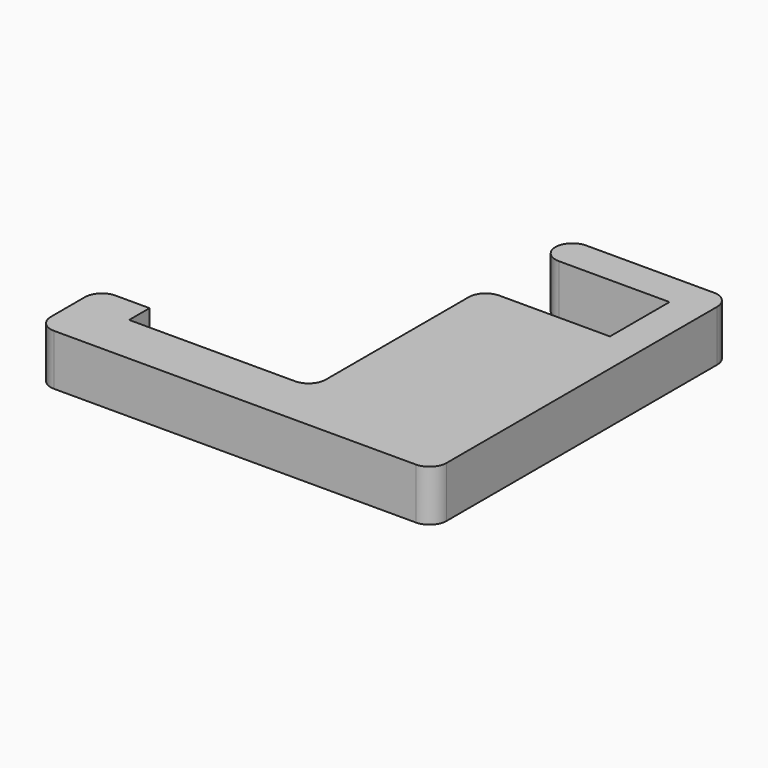
from build123d import *

# Parameters (mm, degrees)
F1_DEPTH = 12
F2_R     = 3.99999


# Not quite as in the source:
# - a fillet or chamfer is up to 0.001 mm smaller than in the source, because OpenCascade refuses the exact size
# - a feature names something its author has since deleted; it is built from what else it names


with BuildPart() as f1:
    # F0 (on Top) → F1 (new body)
    with BuildSketch(Plane.XY):
        Polygon((38, 0), (0, 0), (0, -8), (30, -8), (30, -25.5), (0, -25.5), (0, -75.5), (-43, -75.5), (-43, -69.5), (-55, -69.5), (-55, -87.5), (38, -87.5), align=None)
    extrude(amount=F1_DEPTH)

    # F2 (radius 4 in the source; OpenCascade refuses exactly that, so slightly less here)
    f2_edges = [f1.edges().sort_by_distance(p)[0] for p in [
        (0, -25.5, 6),
        (0, -8, 6),
        (38, 0, 6),
        (38, -87.5, 6),
        (0, 0, 6),
        (-55, -69.5, 6),
        (0, -75.5, 6),
        (-55, -87.5, 6),
    ]]
    fillet(f2_edges, radius=F2_R)


solid = f1.part
